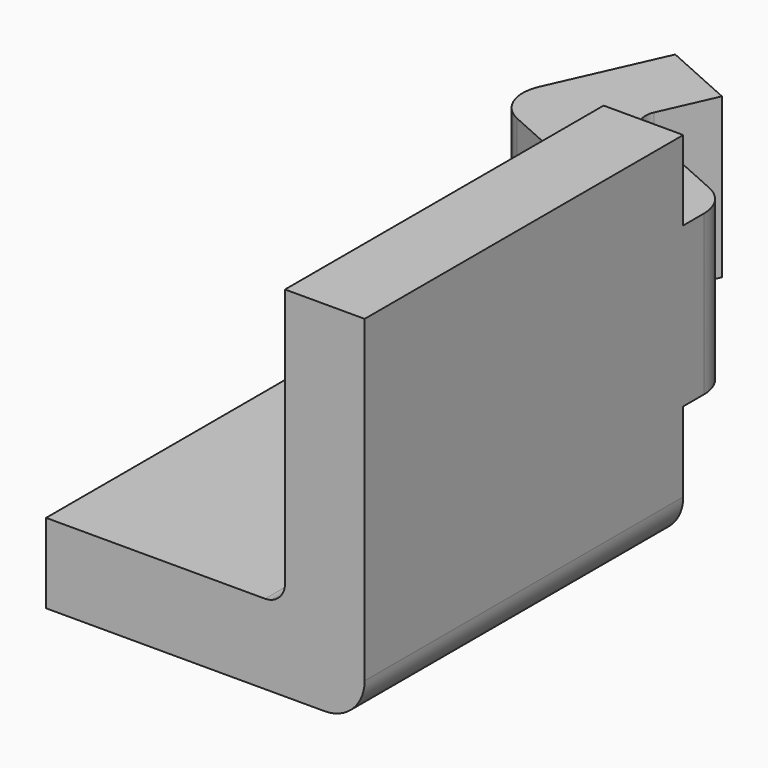
from build123d import *

# Parameters (mm, degrees)
F0_W     = 0.2
F0_H     = 0.7
F1_DEPTH = 1
F3_DEPTH = 0.9
F5_DEPTH = 0.2
F7_DEPTH = 0.3
F8_R     = 0.05
F9_R     = 0.1


with BuildPart() as f1:
    # F0 (on Front) → F1 (new body)
    with BuildSketch(Plane.XZ):
        Polygon((0.2, 0.1), (-0.4, 0.1), (-0.4, -0.1), (0.4, -0.1), (0.4, 0.1), align=None)
        with Locations((0.3, 0.45)):
            Rectangle(F0_W, F0_H)
    extrude(amount=F1_DEPTH)

    # F2 (on face) → F3 (join)
    with BuildSketch(Plane.XY.offset(0.8)):
        Polygon((-0.0658778079, 0.5573172671), (-0.1476107508, 0.3747803502), (0.0349261661, 0.2930474073), (0.116659109, 0.4755843242), align=None)
        Polygon((-0.2293436937, 0.1922434332), (0.2, 0), (0.4, 0), (0.4, 0.1295815215), (0.0349261661, 0.2930474073), (-0.1476107508, 0.3747803502), align=None)
    extrude(amount=-F3_DEPTH)

    # F4 (on face) → F5 (cut)
    with BuildSketch(Plane.XY.offset(0.8)):
        Polygon((0.2, 0), (0.4, 0), (0.4, 0.1295815215), (0.0349261661, 0.2930474073), (0.116659109, 0.4755843242), (-0.0658778079, 0.5573172671), (-0.2293436937, 0.1922434332), align=None)
    extrude(amount=-F5_DEPTH, mode=Mode.SUBTRACT)

    # F6 (on face) → F7 (cut)
    with BuildSketch(Plane(origin=(0, 0, -0.1), x_dir=(1, 0, 0), z_dir=(0, 0, -1))):
        Polygon((0.4, -0.1295815215), (0.4, 0), (0.2, 0), (-0.2293436937, -0.1922434332), (-0.0658778079, -0.5573172671), (0.116659109, -0.4755843242), (0.0349261661, -0.2930474073), align=None)
    extrude(amount=-F7_DEPTH, mode=Mode.SUBTRACT)

    # F8
    f8_edges = [f1.edges().sort_by_distance(p)[0] for p in [
        (0.034926, 0.293047, 0.4),
        (0.2, 0, 0.4),
        (0.2, -0.5, 0.1),
    ]]
    fillet(f8_edges, radius=F8_R)

    # F9
    f9_edges = [f1.edges().sort_by_distance(p)[0] for p in [
        (0.4, -0.5, -0.1),
        (-0.229344, 0.192243, 0.4),
        (0.4, 0.129582, 0.4),
    ]]
    fillet(f9_edges, radius=F9_R)


solid = f1.part
